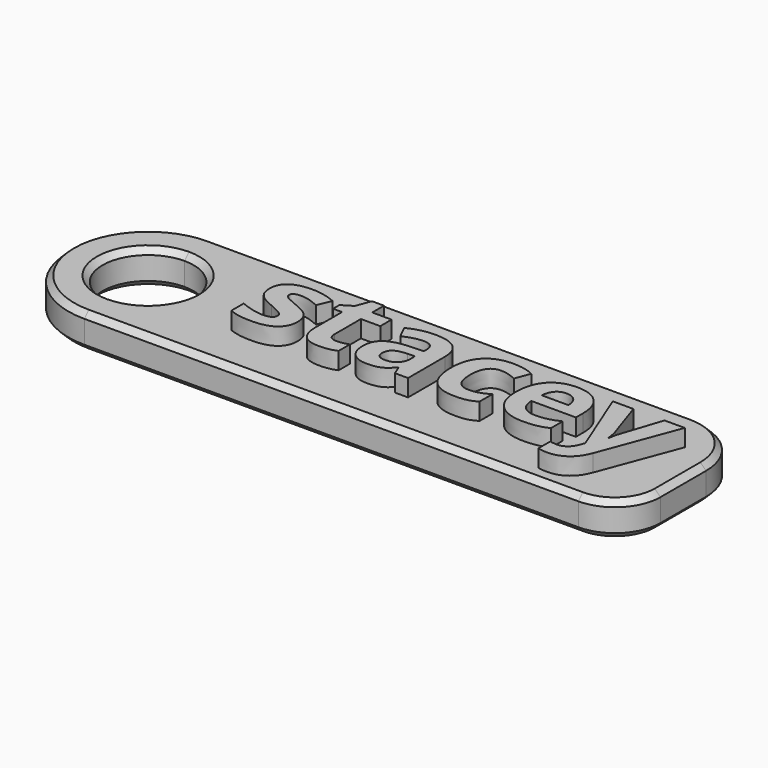
from build123d import *

# Parameters (mm, degrees)
F0_TEXT_SIZE = 11.1111111111
F1_DEPTH     = 3
F2_DEPTH     = 4.5
F3_SIZE      = 0.5


# Not quite as in the source:
# - a feature names something its author has since deleted; it is built from what else it names
# - Text() gives the source's letters only with a copy of the font that has no kerning and outlines rounded to 1/6400 em; it was checked with that copy


with BuildPart() as f1:
    # F0 (on Top) → F1 (new body)
    with BuildSketch(Plane.XY):
        with BuildLine():
            Line((42.3767361111, 7), (0, 7))
            ThreePointArc((0, 7), (4.9497474683, 4.9497474683), (7, 0))
            ThreePointArc((7, 0), (4.9497474683, -4.9497474683), (0, -7))
            Line((0, -7), (43.3767361111, -7))
            ThreePointArc((43.3767361111, -7), (46.2051632359, -5.8284271247), (47.3767361111, -3))
            Line((47.3767361111, -3), (47.3767361111, 2))
            ThreePointArc((47.3767361111, 2), (45.912270017, 5.5355339059), (42.3767361111, 7))
        make_face()
        with BuildLine():
            Line((40.7447916667, -2.9565972222), (38.3350694444, 3.0659722222))
            Line((38.3350694444, 3.0659722222), (40.1475694444, 3.0659722222))
            Line((40.1475694444, 3.0659722222), (41.2916666667, -0.3472222222))
            add(Edge.make_bspline(
                [(41.2916666667, -0.3472222222), (41.4392361111, -0.7916666667), (41.4930555556, -1.3993055556)],
                knots=[0, 0, 0, 1, 1, 1], degree=2))
            Line((41.4930555556, -1.3993055556), (41.5260416667, -1.3993055556))
            add(Edge.make_bspline(
                [(41.5260416667, -1.3993055556), (41.5850694444, -0.8402777778), (41.7586805556, -0.3472222222)],
                knots=[0, 0, 0, 1, 1, 1], degree=2))
            Line((41.7586805556, -0.3472222222), (42.8819444444, 3.0659722222))
            Line((42.8819444444, 3.0659722222), (44.65625, 3.0659722222))
            Line((44.65625, 3.0659722222), (42.0902777778, -3.7760416667))
            add(Edge.make_bspline(
                [(42.0902777778, -3.7760416667), (41.7361111111, -4.7256944444), (41.0824652778, -5.1979166667)],
                knots=[0, 0, 0, 1, 1, 1], degree=2))
            add(Edge.make_bspline(
                [(41.0824652778, -5.1979166667), (40.4288194444, -5.6701388889), (39.5555555556, -5.6701388889)],
                knots=[0, 0, 0, 1, 1, 1], degree=2))
            add(Edge.make_bspline(
                [(39.5555555556, -5.6701388889), (39.1267361111, -5.6701388889), (38.7152777778, -5.5763888889)],
                knots=[0, 0, 0, 1, 1, 1], degree=2))
            Line((38.7152777778, -5.5763888889), (38.7152777778, -4.2638888889))
            add(Edge.make_bspline(
                [(38.7152777778, -4.2638888889), (39.0138888889, -4.3350694444), (39.3663194444, -4.3350694444)],
                knots=[0, 0, 0, 1, 1, 1], degree=2))
            add(Edge.make_bspline(
                [(39.3663194444, -4.3350694444), (39.8055555556, -4.3350694444), (40.1336805556, -4.0659722222)],
                knots=[0, 0, 0, 1, 1, 1], degree=2))
            add(Edge.make_bspline(
                [(40.1336805556, -4.0659722222), (40.4618055556, -3.796875), (40.6458333333, -3.2552083333)],
                knots=[0, 0, 0, 1, 1, 1], degree=2))
            Line((40.6458333333, -3.2552083333), (40.7447916667, -2.9565972222))
        make_face(mode=Mode.SUBTRACT)
        with BuildLine():
            add(Edge.make_bspline(
                [(13.9427083333, -0.4227430556), (14.1006944444, -0.7482638889), (14.1006944444, -1.1979166667)],
                knots=[0, 0, 0, 1, 1, 1], degree=2))
            add(Edge.make_bspline(
                [(14.1006944444, -1.1979166667), (14.1006944444, -2.1319444444), (13.4522569444, -2.6206597222)],
                knots=[0, 0, 0, 1, 1, 1], degree=2))
            add(Edge.make_bspline(
                [(13.4522569444, -2.6206597222), (12.8038194444, -3.109375), (11.5121527778, -3.109375)],
                knots=[0, 0, 0, 1, 1, 1], degree=2))
            add(Edge.make_bspline(
                [(11.5121527778, -3.109375), (10.8506944444, -3.109375), (10.3836805556, -3.0190972222)],
                knots=[0, 0, 0, 1, 1, 1], degree=2))
            add(Edge.make_bspline(
                [(10.3836805556, -3.0190972222), (9.9166666667, -2.9288194444), (9.5104166667, -2.7552083333)],
                knots=[0, 0, 0, 1, 1, 1], degree=2))
            Line((9.5104166667, -2.7552083333), (9.5104166667, -1.3888888889))
            add(Edge.make_bspline(
                [(9.5104166667, -1.3888888889), (9.9704861111, -1.6059027778), (10.5486111111, -1.7526041667)],
                knots=[0, 0, 0, 1, 1, 1], degree=2))
            add(Edge.make_bspline(
                [(10.5486111111, -1.7526041667), (11.1267361111, -1.8993055556), (11.5659722222, -1.8993055556)],
                knots=[0, 0, 0, 1, 1, 1], degree=2))
            add(Edge.make_bspline(
                [(11.5659722222, -1.8993055556), (12.4670138889, -1.8993055556), (12.4670138889, -1.3784722222)],
                knots=[0, 0, 0, 1, 1, 1], degree=2))
            add(Edge.make_bspline(
                [(12.4670138889, -1.3784722222), (12.4670138889, -1.1822916667), (12.3472222222, -1.0598958333)],
                knots=[0, 0, 0, 1, 1, 1], degree=2))
            add(Edge.make_bspline(
                [(12.3472222222, -1.0598958333), (12.2274305556, -0.9375), (11.9348958333, -0.7829861111)],
                knots=[0, 0, 0, 1, 1, 1], degree=2))
            add(Edge.make_bspline(
                [(11.9348958333, -0.7829861111), (11.6423611111, -0.6284722222), (11.1545138889, -0.4236111111)],
                knots=[0, 0, 0, 1, 1, 1], degree=2))
            add(Edge.make_bspline(
                [(11.1545138889, -0.4236111111), (10.4548611111, -0.1302083333), (10.1258680556, 0.1197916667)],
                knots=[0, 0, 0, 1, 1, 1], degree=2))
            add(Edge.make_bspline(
                [(10.1258680556, 0.1197916667), (9.796875, 0.3697916667), (9.6484375, 0.6927083333)],
                knots=[0, 0, 0, 1, 1, 1], degree=2))
            add(Edge.make_bspline(
                [(9.6484375, 0.6927083333), (9.5, 1.015625), (9.5, 1.4861111111)],
                knots=[0, 0, 0, 1, 1, 1], degree=2))
            add(Edge.make_bspline(
                [(9.5, 1.4861111111), (9.5, 2.2951388889), (10.1258680556, 2.7369791667)],
                knots=[0, 0, 0, 1, 1, 1], degree=2))
            add(Edge.make_bspline(
                [(10.1258680556, 2.7369791667), (10.7517361111, 3.1788194444), (11.9027777778, 3.1788194444)],
                knots=[0, 0, 0, 1, 1, 1], degree=2))
            add(Edge.make_bspline(
                [(11.9027777778, 3.1788194444), (12.9982638889, 3.1788194444), (14.0347222222, 2.7013888889)],
                knots=[0, 0, 0, 1, 1, 1], degree=2))
            Line((14.0347222222, 2.7013888889), (13.5364583333, 1.5086805556))
            add(Edge.make_bspline(
                [(13.5364583333, 1.5086805556), (13.0798611111, 1.703125), (12.6840277778, 1.828125)],
                knots=[0, 0, 0, 1, 1, 1], degree=2))
            add(Edge.make_bspline(
                [(12.6840277778, 1.828125), (12.2881944444, 1.953125), (11.875, 1.953125)],
                knots=[0, 0, 0, 1, 1, 1], degree=2))
            add(Edge.make_bspline(
                [(11.875, 1.953125), (11.1423611111, 1.953125), (11.1423611111, 1.5572916667)],
                knots=[0, 0, 0, 1, 1, 1], degree=2))
            add(Edge.make_bspline(
                [(11.1423611111, 1.5572916667), (11.1423611111, 1.3350694444), (11.3784722222, 1.171875)],
                knots=[0, 0, 0, 1, 1, 1], degree=2))
            add(Edge.make_bspline(
                [(11.3784722222, 1.171875), (11.6145833333, 1.0086805556), (12.4131944444, 0.6892361111)],
                knots=[0, 0, 0, 1, 1, 1], degree=2))
            add(Edge.make_bspline(
                [(12.4131944444, 0.6892361111), (13.1232638889, 0.4010416667), (13.4539930556, 0.1519097222)],
                knots=[0, 0, 0, 1, 1, 1], degree=2))
            add(Edge.make_bspline(
                [(13.4539930556, 0.1519097222), (13.7847222222, -0.0972222222), (13.9427083333, -0.4227430556)],
                knots=[0, 0, 0, 1, 1, 1], degree=2))
        make_face(mode=Mode.SUBTRACT)
        with BuildLine():
            add(Edge.make_bspline(
                [(17.421875, -1.6215277778), (17.6197916667, -1.7899305556), (17.9461805556, -1.7899305556)],
                knots=[0, 0, 0, 1, 1, 1], degree=2))
            add(Edge.make_bspline(
                [(17.9461805556, -1.7899305556), (18.3802083333, -1.7899305556), (18.9878472222, -1.6006944444)],
                knots=[0, 0, 0, 1, 1, 1], degree=2))
            Line((18.9878472222, -1.6006944444), (18.9878472222, -2.8315972222))
            add(Edge.make_bspline(
                [(18.9878472222, -2.8315972222), (18.3697916667, -3.109375), (17.46875, -3.109375)],
                knots=[0, 0, 0, 1, 1, 1], degree=2))
            add(Edge.make_bspline(
                [(17.46875, -3.109375), (16.4756944444, -3.109375), (16.0225694444, -2.6067708333)],
                knots=[0, 0, 0, 1, 1, 1], degree=2))
            add(Edge.make_bspline(
                [(16.0225694444, -2.6067708333), (15.5694444444, -2.1041666667), (15.5694444444, -1.1006944444)],
                knots=[0, 0, 0, 1, 1, 1], degree=2))
            Line((15.5694444444, -1.1006944444), (15.5694444444, 1.8229166667))
            Line((15.5694444444, 1.8229166667), (14.7777777778, 1.8229166667))
            Line((14.7777777778, 1.8229166667), (14.7777777778, 2.5225694444))
            Line((14.7777777778, 2.5225694444), (15.6892361111, 3.0763888889))
            Line((15.6892361111, 3.0763888889), (16.1666666667, 4.3576388889))
            Line((16.1666666667, 4.3576388889), (17.2239583333, 4.3576388889))
            Line((17.2239583333, 4.3576388889), (17.2239583333, 3.0659722222))
            Line((17.2239583333, 3.0659722222), (18.921875, 3.0659722222))
            Line((18.921875, 3.0659722222), (18.921875, 1.8229166667))
            Line((18.921875, 1.8229166667), (17.2239583333, 1.8229166667))
            Line((17.2239583333, 1.8229166667), (17.2239583333, -1.1006944444))
            add(Edge.make_bspline(
                [(17.2239583333, -1.1006944444), (17.2239583333, -1.453125), (17.421875, -1.6215277778)],
                knots=[0, 0, 0, 1, 1, 1], degree=2))
        make_face(mode=Mode.SUBTRACT)
        with BuildLine():
            Line((25.2204861111, -3), (24.0659722222, -3))
            Line((24.0659722222, -3), (23.7447916667, -2.1753472222))
            Line((23.7447916667, -2.1753472222), (23.7013888889, -2.1753472222))
            add(Edge.make_bspline(
                [(23.7013888889, -2.1753472222), (23.2847222222, -2.7013888889), (22.8420138889, -2.9053819444)],
                knots=[0, 0, 0, 1, 1, 1], degree=2))
            add(Edge.make_bspline(
                [(22.8420138889, -2.9053819444), (22.3993055556, -3.109375), (21.6892361111, -3.109375)],
                knots=[0, 0, 0, 1, 1, 1], degree=2))
            add(Edge.make_bspline(
                [(21.6892361111, -3.109375), (20.8159722222, -3.109375), (20.3142361111, -2.609375)],
                knots=[0, 0, 0, 1, 1, 1], degree=2))
            add(Edge.make_bspline(
                [(20.3142361111, -2.609375), (19.8125, -2.109375), (19.8125, -1.1875)],
                knots=[0, 0, 0, 1, 1, 1], degree=2))
            add(Edge.make_bspline(
                [(19.8125, -1.1875), (19.8125, -0.2222222222), (20.4878472222, 0.2361111111)],
                knots=[0, 0, 0, 1, 1, 1], degree=2))
            add(Edge.make_bspline(
                [(20.4878472222, 0.2361111111), (21.1631944444, 0.6944444444), (22.5243055556, 0.7430555556)],
                knots=[0, 0, 0, 1, 1, 1], degree=2))
            Line((22.5243055556, 0.7430555556), (23.578125, 0.7760416667))
            Line((23.578125, 0.7760416667), (23.578125, 1.0416666667))
            add(Edge.make_bspline(
                [(23.578125, 1.0416666667), (23.578125, 1.9635416667), (22.6336805556, 1.9635416667)],
                knots=[0, 0, 0, 1, 1, 1], degree=2))
            add(Edge.make_bspline(
                [(22.6336805556, 1.9635416667), (21.90625, 1.9635416667), (20.9236111111, 1.5243055556)],
                knots=[0, 0, 0, 1, 1, 1], degree=2))
            Line((20.9236111111, 1.5243055556), (20.3767361111, 2.6423611111))
            add(Edge.make_bspline(
                [(20.3767361111, 2.6423611111), (21.4236111111, 3.1909722222), (22.6979166667, 3.1909722222)],
                knots=[0, 0, 0, 1, 1, 1], degree=2))
            add(Edge.make_bspline(
                [(22.6979166667, 3.1909722222), (23.9184027778, 3.1909722222), (24.5694444444, 2.6588541667)],
                knots=[0, 0, 0, 1, 1, 1], degree=2))
            add(Edge.make_bspline(
                [(24.5694444444, 2.6588541667), (25.2204861111, 2.1267361111), (25.2204861111, 1.0416666667)],
                knots=[0, 0, 0, 1, 1, 1], degree=2))
            Line((25.2204861111, 1.0416666667), (25.2204861111, -3))
        make_face(mode=Mode.SUBTRACT)
        with BuildLine():
            add(Edge.make_bspline(
                [(30.421875, -3.0112847222), (30.0121527778, -3.109375), (29.3888888889, -3.109375)],
                knots=[0, 0, 0, 1, 1, 1], degree=2))
            add(Edge.make_bspline(
                [(29.3888888889, -3.109375), (26.5572916667, -3.109375), (26.5572916667, 0)],
                knots=[0, 0, 0, 1, 1, 1], degree=2))
            add(Edge.make_bspline(
                [(26.5572916667, 0), (26.5572916667, 1.546875), (27.3272569444, 2.3628472222)],
                knots=[0, 0, 0, 1, 1, 1], degree=2))
            add(Edge.make_bspline(
                [(27.3272569444, 2.3628472222), (28.0972222222, 3.1788194444), (29.5347222222, 3.1788194444)],
                knots=[0, 0, 0, 1, 1, 1], degree=2))
            add(Edge.make_bspline(
                [(29.5347222222, 3.1788194444), (30.5868055556, 3.1788194444), (31.4236111111, 2.7673611111)],
                knots=[0, 0, 0, 1, 1, 1], degree=2))
            Line((31.4236111111, 2.7673611111), (30.9340277778, 1.4861111111))
            add(Edge.make_bspline(
                [(30.9340277778, 1.4861111111), (30.5434027778, 1.6440972222), (30.2074652778, 1.7447916667)],
                knots=[0, 0, 0, 1, 1, 1], degree=2))
            add(Edge.make_bspline(
                [(30.2074652778, 1.7447916667), (29.8715277778, 1.8454861111), (29.5347222222, 1.8454861111)],
                knots=[0, 0, 0, 1, 1, 1], degree=2))
            add(Edge.make_bspline(
                [(29.5347222222, 1.8454861111), (28.2430555556, 1.8454861111), (28.2430555556, 0.0104166667)],
                knots=[0, 0, 0, 1, 1, 1], degree=2))
            add(Edge.make_bspline(
                [(28.2430555556, 0.0104166667), (28.2430555556, -1.7690972222), (29.5347222222, -1.7690972222)],
                knots=[0, 0, 0, 1, 1, 1], degree=2))
            add(Edge.make_bspline(
                [(29.5347222222, -1.7690972222), (30.0121527778, -1.7690972222), (30.4192708333, -1.6414930556)],
                knots=[0, 0, 0, 1, 1, 1], degree=2))
            add(Edge.make_bspline(
                [(30.4192708333, -1.6414930556), (30.8263888889, -1.5138888889), (31.2326388889, -1.2413194444)],
                knots=[0, 0, 0, 1, 1, 1], degree=2))
            Line((31.2326388889, -1.2413194444), (31.2326388889, -2.6579861111))
            add(Edge.make_bspline(
                [(31.2326388889, -2.6579861111), (30.8315972222, -2.9131944444), (30.421875, -3.0112847222)],
                knots=[0, 0, 0, 1, 1, 1], degree=2))
        make_face(mode=Mode.SUBTRACT)
        with BuildLine():
            add(Edge.make_bspline(
                [(36.5885416667, -3.0034722222), (36.0954861111, -3.109375), (35.3836805556, -3.109375)],
                knots=[0, 0, 0, 1, 1, 1], degree=2))
            add(Edge.make_bspline(
                [(35.3836805556, -3.109375), (33.9201388889, -3.109375), (33.0954861111, -2.3003472222)],
                knots=[0, 0, 0, 1, 1, 1], degree=2))
            add(Edge.make_bspline(
                [(33.0954861111, -2.3003472222), (32.2708333333, -1.4913194444), (32.2708333333, -0.0104166667)],
                knots=[0, 0, 0, 1, 1, 1], degree=2))
            add(Edge.make_bspline(
                [(32.2708333333, -0.0104166667), (32.2708333333, 1.5138888889), (33.0329861111, 2.3463541667)],
                knots=[0, 0, 0, 1, 1, 1], degree=2))
            add(Edge.make_bspline(
                [(33.0329861111, 2.3463541667), (33.7951388889, 3.1788194444), (35.140625, 3.1788194444)],
                knots=[0, 0, 0, 1, 1, 1], degree=2))
            add(Edge.make_bspline(
                [(35.140625, 3.1788194444), (36.4253472222, 3.1788194444), (37.1414930556, 2.4470486111)],
                knots=[0, 0, 0, 1, 1, 1], degree=2))
            add(Edge.make_bspline(
                [(37.1414930556, 2.4470486111), (37.8576388889, 1.7152777778), (37.8576388889, 0.4236111111)],
                knots=[0, 0, 0, 1, 1, 1], degree=2))
            Line((37.8576388889, 0.4236111111), (37.8576388889, -0.3802083333))
            Line((37.8576388889, -0.3802083333), (33.9461805556, -0.3802083333))
            add(Edge.make_bspline(
                [(33.9461805556, -0.3802083333), (33.9739583333, -1.0850694444), (34.3645833333, -1.4809027778)],
                knots=[0, 0, 0, 1, 1, 1], degree=2))
            add(Edge.make_bspline(
                [(34.3645833333, -1.4809027778), (34.7552083333, -1.8767361111), (35.4600694444, -1.8767361111)],
                knots=[0, 0, 0, 1, 1, 1], degree=2))
            add(Edge.make_bspline(
                [(35.4600694444, -1.8767361111), (36.0086805556, -1.8767361111), (36.4965277778, -1.7630208333)],
                knots=[0, 0, 0, 1, 1, 1], degree=2))
            add(Edge.make_bspline(
                [(36.4965277778, -1.7630208333), (36.984375, -1.6493055556), (37.515625, -1.3993055556)],
                knots=[0, 0, 0, 1, 1, 1], degree=2))
            Line((37.515625, -1.3993055556), (37.515625, -2.6805555556))
            add(Edge.make_bspline(
                [(37.515625, -2.6805555556), (37.0815972222, -2.8975694444), (36.5885416667, -3.0034722222)],
                knots=[0, 0, 0, 1, 1, 1], degree=2))
        make_face(mode=Mode.SUBTRACT)
        with BuildLine():
            ThreePointArc((0, -4), (-4, 0), (0, 4))
            Line((0, 4), (0, 7))
            ThreePointArc((0, 7), (-7, 0), (0, -7))
            Line((0, -7), (0, -4))
        make_face()
        with BuildLine():
            ThreePointArc((0, 4), (2.8284271247, 2.8284271247), (4, 0))
            ThreePointArc((4, 0), (2.8284271247, -2.8284271247), (0, -4))
            Line((0, -4), (0, -7))
            ThreePointArc((0, -7), (4.9497474683, -4.9497474683), (7, 0))
            ThreePointArc((7, 0), (4.9497474683, 4.9497474683), (0, 7))
            Line((0, 7), (0, 4))
        make_face()
        with Locations((9, -3)):
            Text('stacey', F0_TEXT_SIZE, font='Open Sans', font_style=FontStyle.BOLD, text_align=(TextAlign.LEFT, TextAlign.BOTTOM))
        with BuildLine():
            Line((23.578125, -0.6892361111), (23.578125, -0.1892361111))
            Line((23.578125, -0.1892361111), (22.9375, -0.2118055556))
            add(Edge.make_bspline(
                [(22.9375, -0.2118055556), (22.2152777778, -0.2326388889), (21.8628472222, -0.4713541667)],
                knots=[0, 0, 0, 1, 1, 1], degree=2))
            add(Edge.make_bspline(
                [(21.8628472222, -0.4713541667), (21.5104166667, -0.7100694444), (21.5104166667, -1.1979166667)],
                knots=[0, 0, 0, 1, 1, 1], degree=2))
            add(Edge.make_bspline(
                [(21.5104166667, -1.1979166667), (21.5104166667, -1.8993055556), (22.3125, -1.8993055556)],
                knots=[0, 0, 0, 1, 1, 1], degree=2))
            add(Edge.make_bspline(
                [(22.3125, -1.8993055556), (22.8888888889, -1.8993055556), (23.2335069444, -1.5677083333)],
                knots=[0, 0, 0, 1, 1, 1], degree=2))
            add(Edge.make_bspline(
                [(23.2335069444, -1.5677083333), (23.578125, -1.2361111111), (23.578125, -0.6892361111)],
                knots=[0, 0, 0, 1, 1, 1], degree=2))
        make_face()
        with BuildLine():
            add(Edge.make_bspline(
                [(35.9861111111, 1.6684027778), (35.6770833333, 2.0017361111), (35.1510416667, 2.0017361111)],
                knots=[0, 0, 0, 1, 1, 1], degree=2))
            add(Edge.make_bspline(
                [(35.1510416667, 2.0017361111), (34.625, 2.0017361111), (34.3263888889, 1.6684027778)],
                knots=[0, 0, 0, 1, 1, 1], degree=2))
            add(Edge.make_bspline(
                [(34.3263888889, 1.6684027778), (34.0277777778, 1.3350694444), (33.984375, 0.7222222222)],
                knots=[0, 0, 0, 1, 1, 1], degree=2))
            Line((33.984375, 0.7222222222), (36.3072916667, 0.7222222222))
            add(Edge.make_bspline(
                [(36.3072916667, 0.7222222222), (36.2951388889, 1.3350694444), (35.9861111111, 1.6684027778)],
                knots=[0, 0, 0, 1, 1, 1], degree=2))
        make_face()
    extrude(amount=F1_DEPTH)

    # F0 (on Top) → F2 (join)
    with BuildSketch(Plane.XY):
        with Locations((9, -3)):
            Text('stacey', F0_TEXT_SIZE, font='Open Sans', font_style=FontStyle.BOLD, text_align=(TextAlign.LEFT, TextAlign.BOTTOM))
    extrude(amount=F2_DEPTH)

    # F3
    f3_edges = [f1.edges().sort_by_distance(p)[0] for p in [
        (-4, 0, 0),
        (47.376736, -0.5, 0),
        (47.376736, -0.5, 3),
        (-4, 0, 3),
    ]]
    chamfer(f3_edges, length=F3_SIZE)


solid = f1.part
